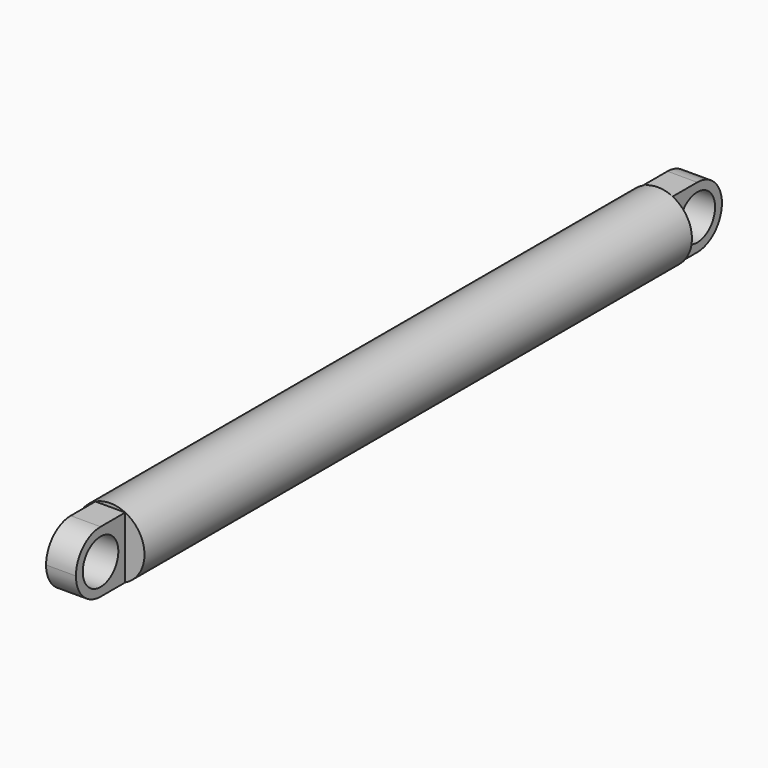
from build123d import *

# Parameters (mm, degrees)
F0_W      = 5
F0_H      = 100
F2_W      = 4.3588989435
F2_H      = 9
F3_DEPTH  = 9
F4_R      = 3.25
F5_DEPTH  = 5
F6_R      = 4.49999
F7_W      = 4.3588989435
F7_H      = 9
F8_DEPTH  = 9
F9_R      = 3.25
F10_DEPTH = 5
F11_R     = 4.49999


# Not quite as in the source:
# - a fillet or chamfer is up to 0.001 mm smaller than in the source, because OpenCascade refuses the exact size


with BuildPart() as f1:
    # F0 (on Top) → F1 (revolve)
    with BuildSketch(Plane.XY):
        with Locations((-2.5, 50)):
            Rectangle(F0_W, F0_H)
    revolve(axis=Axis((0, 50, 0), (0, -1, 0)))

    # F2 (on face) → F3 (join)
    with BuildSketch(Plane.XZ):
        Rectangle(F2_W, F2_H)
    extrude(amount=F3_DEPTH)

    # F4 (on face) → F5 (cut)
    with BuildSketch(Plane.YZ.offset(2.1794494718)):
        with Locations((-4.5, 0)):
            Circle(F4_R)
    extrude(amount=-F5_DEPTH, mode=Mode.SUBTRACT)

    # F6 (radius 4.5 in the source; OpenCascade refuses exactly that, so slightly less here)
    f6_edges = [f1.edges().sort_by_distance(p)[0] for p in [
        (0, -9, 4.5),
        (0, -9, -4.5),
    ]]
    fillet(f6_edges, radius=F6_R)

    # F7 (on face) → F8 (join)
    with BuildSketch(Plane(origin=(0, 100, 0), x_dir=(-1, 0, 0), z_dir=(0, 1, 0))):
        Rectangle(F7_W, F7_H)
    extrude(amount=F8_DEPTH)

    # F9 (on face) → F10 (cut)
    with BuildSketch(Plane(origin=(-2.1794494718, 0, 0), x_dir=(0, -1, 0), z_dir=(-1, 0, 0))):
        with Locations((-104.5, 0)):
            Circle(F9_R)
    extrude(amount=-F10_DEPTH, mode=Mode.SUBTRACT)

    # F11 (radius 4.5 in the source; OpenCascade refuses exactly that, so slightly less here)
    f11_edges = [f1.edges().sort_by_distance(p)[0] for p in [
        (0, 109, 4.5),
        (0, 109, -4.5),
    ]]
    fillet(f11_edges, radius=F11_R)


solid = f1.part
